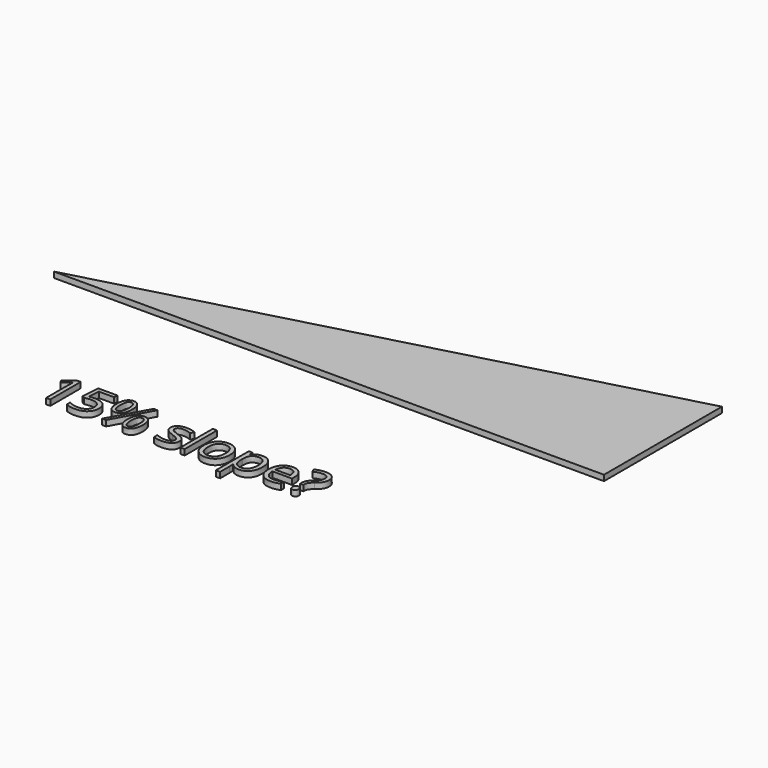
from build123d import *

# Parameters (mm, degrees)
F0_TEXT_SIZE = 237.651500437
F1_DEPTH     = 25.4


# Not quite as in the source:
# - Text() gives the source's letters only with a copy of the font that has no kerning and outlines rounded to 1/6400 em; it was checked with that copy


with BuildPart() as f1:
    # F0 (on Top) → F1 (new body)
    with BuildSketch(Plane.XY):
        Polygon((1434.1485587677, 657.4003745604), (-1019.3030400065, 0), (1434.1485587677, 0), align=None)
        with Locations((-508.8127851486, -761.0937356949)):
            Text('15% slope?', F0_TEXT_SIZE, font='Open Sans', text_align=(TextAlign.LEFT, TextAlign.BOTTOM))
    extrude(amount=F1_DEPTH)


solid = f1.part
